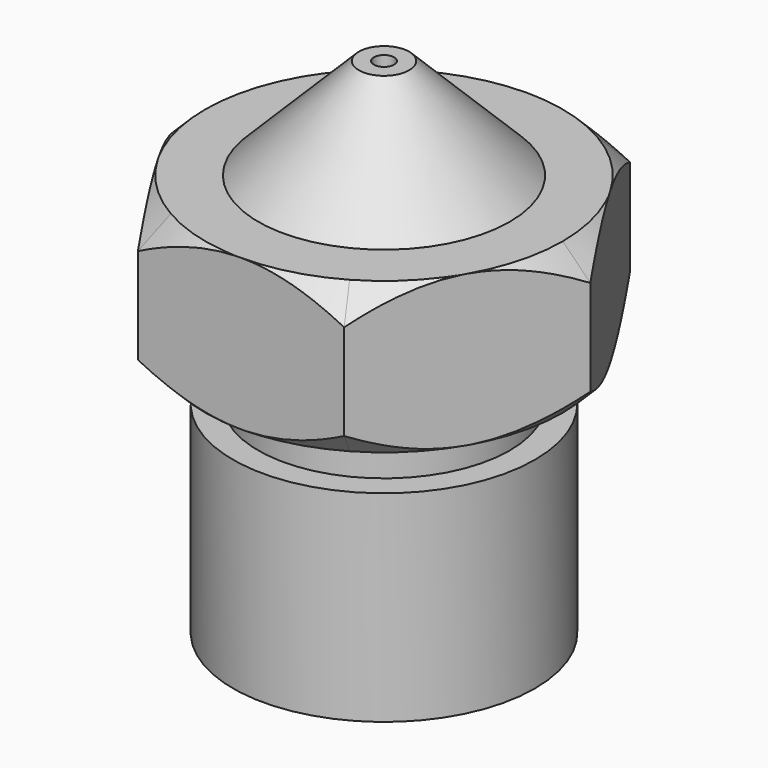
from build123d import *

# Parameters (mm, degrees)
F0_R      = 2.5
F0_R_2    = 0.2
F1_DEPTH  = 3
F2_SIZE   = 0.54919
F3_DEPTH  = 3.001
F4_DEPTH  = 5
F5_SIZE   = 1.99999
F6_DEPTH  = 1
F7_R      = 3
F7_R_2    = 2.5
F7_R_3    = 0.2
F8_DEPTH  = 4
F9_R      = 1
F9_R_2    = 0.2
F10_DEPTH = 6
F11_SIZE  = 0.79999


# Not quite as in the source:
# - a fillet or chamfer is up to 0.001 mm smaller than in the source, because OpenCascade refuses the exact size


with BuildPart() as f1:
    # F0 (on Top) → F1 (new body)
    with BuildSketch(Plane.XY):
        Polygon((2.0495934556, 3.55), (-2.0495934556, 3.55), (-4.0991869112, 0), (-2.0495934556, -3.55), (2.0495934556, -3.55), (4.0991869112, 0), align=None)
        Circle(F0_R, mode=Mode.SUBTRACT)
        with BuildLine():
            Line((-4.0991869112, 0), (-2.0495934556, 3.55))
            ThreePointArc((-2.0495934556, 3.55), (-3.55, 2.0495934556), (-4.0991869112, 0))
        make_face()
        with BuildLine():
            Line((-2.0495934556, -3.55), (-4.0991869112, 0))
            ThreePointArc((-4.0991869112, 0), (-3.55, -2.0495934556), (-2.0495934556, -3.55))
        make_face()
        with BuildLine():
            ThreePointArc((2.0495934556, 3.55), (0, 4.0991869112), (-2.0495934556, 3.55))
            Line((-2.0495934556, 3.55), (2.0495934556, 3.55))
        make_face()
        with BuildLine():
            ThreePointArc((4.0991869112, 0), (3.55, 2.0495934556), (2.0495934556, 3.55))
            Line((2.0495934556, 3.55), (4.0991869112, 0))
        make_face()
        with BuildLine():
            ThreePointArc((2.0495934556, -3.55), (3.55, -2.0495934556), (4.0991869112, 0))
            Line((4.0991869112, 0), (2.0495934556, -3.55))
        make_face()
        with BuildLine():
            Line((2.0495934556, -3.55), (-2.0495934556, -3.55))
            ThreePointArc((-2.0495934556, -3.55), (0, -4.0991869112), (2.0495934556, -3.55))
        make_face()
        Circle(F0_R)
        Circle(F0_R_2, mode=Mode.SUBTRACT)
    extrude(amount=F1_DEPTH)

    # F2
    f2_edges = [f1.edges().sort_by_distance(p)[0] for p in [
        (2.049593, 3.55, 3),
        (2.049593, 3.55, 0),
    ]]
    chamfer(f2_edges, length=F2_SIZE)

    # F0 (on Top) → F3 (cut, through all)
    with BuildSketch(Plane.XY):
        with BuildLine():
            Line((2.0495934556, -3.55), (-2.0495934556, -3.55))
            ThreePointArc((-2.0495934556, -3.55), (0, -4.0991869112), (2.0495934556, -3.55))
        make_face()
        with BuildLine():
            ThreePointArc((2.0495934556, -3.55), (3.55, -2.0495934556), (4.0991869112, 0))
            Line((4.0991869112, 0), (2.0495934556, -3.55))
        make_face()
        with BuildLine():
            Line((-2.0495934556, -3.55), (-4.0991869112, 0))
            ThreePointArc((-4.0991869112, 0), (-3.55, -2.0495934556), (-2.0495934556, -3.55))
        make_face()
        with BuildLine():
            ThreePointArc((4.0991869112, 0), (3.55, 2.0495934556), (2.0495934556, 3.55))
            Line((2.0495934556, 3.55), (4.0991869112, 0))
        make_face()
        with BuildLine():
            ThreePointArc((2.0495934556, 3.55), (0, 4.0991869112), (-2.0495934556, 3.55))
            Line((-2.0495934556, 3.55), (2.0495934556, 3.55))
        make_face()
        with BuildLine():
            Line((-4.0991869112, 0), (-2.0495934556, 3.55))
            ThreePointArc((-2.0495934556, 3.55), (-3.55, 2.0495934556), (-4.0991869112, 0))
        make_face()
    extrude(amount=F3_DEPTH, mode=Mode.SUBTRACT)

    # F0 (on Top) → F4 (join)
    with BuildSketch(Plane.XY):
        Circle(F0_R)
        Circle(F0_R_2, mode=Mode.SUBTRACT)
    extrude(amount=F4_DEPTH)

    # F5 (size 2 in the source; OpenCascade refuses exactly that, so slightly less here)
    f5_edges = [f1.edges().sort_by_distance(p)[0] for p in [
        (-2.5, 0, 5),
    ]]
    chamfer(f5_edges, length=F5_SIZE)

    # F0 (on Top) → F6 (join)
    with BuildSketch(Plane.XY):
        Circle(F0_R)
        Circle(F0_R_2, mode=Mode.SUBTRACT)
    extrude(amount=-F6_DEPTH)

    # F7 (on face) → F8 (join)
    with BuildSketch(Plane(origin=(0, 0, -1), x_dir=(1, 0, 0), z_dir=(0, 0, -1))):
        Circle(F7_R)
        Circle(F7_R_2, mode=Mode.SUBTRACT)
        Circle(F7_R_2)
        Circle(F7_R_3, mode=Mode.SUBTRACT)
    extrude(amount=F8_DEPTH)

    # F9 (on face) → F10 (cut)
    with BuildSketch(Plane(origin=(0, 0, -5), x_dir=(1, 0, 0), z_dir=(0, 0, -1))):
        Circle(F9_R)
        Circle(F9_R_2, mode=Mode.SUBTRACT)
    extrude(amount=-F10_DEPTH, mode=Mode.SUBTRACT)

    # F11 (size 0.8 in the source; OpenCascade refuses exactly that, so slightly less here)
    f11_edges = [f1.edges().sort_by_distance(p)[0] for p in [
        (-1, 0, 1),
    ]]
    chamfer(f11_edges, length=F11_SIZE)


solid = f1.part
